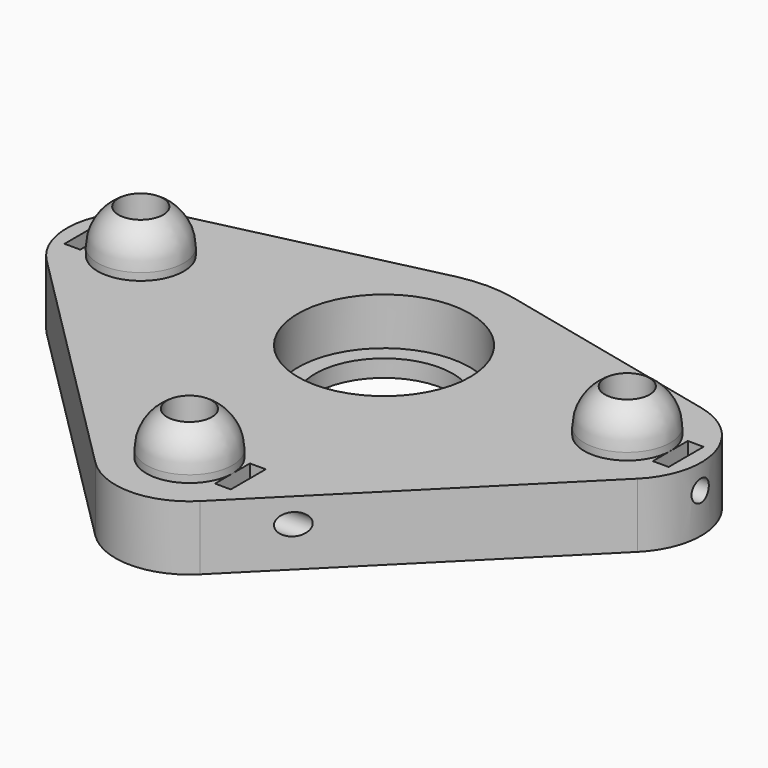
from build123d import *

# Parameters (mm, degrees)
F0_R        = 3.302
F0_R_2      = 12.7
F1_DEPTH    = 9.525
F0_R_3      = 10.16
F2_DEPTH    = 2.54
F5_DEPTH    = 8.636
F6_T1_DEPTH = 2.3368
F6_T3_DEPTH = 2.3368
F6_T5_DEPTH = 2.3368
F3_R        = 6.35
F3_R_2      = 3.302
F7_DEPTH    = 6.35
F11_R       = 1.5875
F12_DEPTH   = 6.35
F9_R        = 1.5875
F13_DEPTH   = 6.35
F10_R       = 1.5875
F14_DEPTH   = 8.382


# Not quite as in the source:
# - a fillet or chamfer that OpenCascade refuses, or shapes differently, is made with other operations: its cross-section is extruded or revolved along the edge and cut away or added
# - a feature names something its author has since deleted; it is built from what else it names


with BuildPart() as f1:
    # F0 (on Top) → F1 (new body)
    with BuildSketch(Plane.XY):
        with BuildLine():
            Line((38.3924752276, 46.5596586637), (4.3105120801, 54.476849111))
            ThreePointArc((4.3105120801, 54.476849111), (0, 54.970934), (-4.3105120801, 54.476849111))
            Line((-4.3105120801, 54.476849111), (-38.3924752276, 46.5596586637))
            ThreePointArc((-38.3924752276, 46.5596586637), (-46.4220600308, 38.9243049052), (-43.6441157783, 28.1978942818))
            Line((-43.6441157783, 28.1978942818), (-7.72300081, -7.7230397182))
            ThreePointArc((-7.72300081, -7.7230397182), (0, -10.922), (7.72300081, -7.7230397182))
            Line((7.72300081, -7.7230397182), (43.6441157783, 28.1978942818))
            ThreePointArc((43.6441157783, 28.1978942818), (46.4220600308, 38.9243049052), (38.3924752276, 46.5596586637))
        make_face()
        Circle(F0_R, mode=Mode.SUBTRACT)
        with Locations((-35.9211149683, 35.920934)):
            Circle(F0_R, mode=Mode.SUBTRACT)
        with Locations((0, 35.920934)):
            Circle(F0_R_2, mode=Mode.SUBTRACT)
        with Locations((35.9211149683, 35.920934)):
            Circle(F0_R, mode=Mode.SUBTRACT)
    extrude(amount=F1_DEPTH)

    # F0 (on Top) → F2 (join)
    with BuildSketch(Plane.XY):
        with Locations((0, 35.920934)):
            Circle(F0_R_2)
        with Locations((0, 35.920934)):
            Circle(F0_R_3, mode=Mode.SUBTRACT)
    extrude(amount=F2_DEPTH)

    # F4 (on face) → F5 (cut)
    with BuildSketch(Plane.XY.offset(9.525)):
        Polygon((-42.2711149683, 32.695134), (-42.2711149683, 35.920934), (-42.2711149683, 39.146734), (-44.6079149683, 39.146734), (-44.6079149683, 32.695134), align=None)
        Polygon((42.2711149683, 39.146734), (42.2711149683, 35.920934), (42.2711149683, 32.695134), (44.6079149683, 32.695134), (44.6079149683, 39.146734), align=None)
        Polygon((6.35, 3.2258), (6.35, 0), (6.35, -3.2258), (8.6868, -3.2258), (8.6868, 3.2258), align=None)
    extrude(amount=-F5_DEPTH, mode=Mode.SUBTRACT)

    # F6: chamfer of 3.175 x 5.499261314 on 6 edges, made by hand

    # F6_s2 → F6_t1 (join)
    with BuildSketch(Plane.YZ.offset(-44.6079149683)):
        Polygon((39.146734, 4.064), (33.647472686, 0.889), (39.146734, 0.889), align=None)
        Polygon((32.695134, 4.064), (38.194395314, 0.889), (32.695134, 0.889), align=None)
    extrude(amount=F6_T1_DEPTH)

    # F6_s4 → F6_t3 (join)
    with BuildSketch(Plane.YZ.offset(6.35)):
        Polygon((3.2258, 4.064), (-2.273461314, 0.889), (3.2258, 0.889), align=None)
        Polygon((-3.2258, 4.064), (2.273461314, 0.889), (-3.2258, 0.889), align=None)
    extrude(amount=F6_T3_DEPTH)

    # F6_s6 → F6_t5 (join)
    with BuildSketch(Plane.YZ.offset(42.2711149683)):
        Polygon((39.146734, 4.064), (33.647472686, 0.889), (39.146734, 0.889), align=None)
        Polygon((32.695134, 4.064), (38.194395314, 0.889), (32.695134, 0.889), align=None)
    extrude(amount=F6_T5_DEPTH)

    # F3 (on face) → F7 (join)
    with BuildSketch(Plane.XY.offset(9.525)):
        with Locations((-35.9211149683, 35.920934)):
            Circle(F3_R)
        with Locations((-35.9211149683, 35.920934)):
            Circle(F3_R_2, mode=Mode.SUBTRACT)
        Circle(F3_R)
        Circle(F3_R_2, mode=Mode.SUBTRACT)
        with Locations((35.9211149683, 35.920934)):
            Circle(F3_R)
        with Locations((35.9211149683, 35.920934)):
            Circle(F3_R_2, mode=Mode.SUBTRACT)
    extrude(amount=F7_DEPTH)

    # F8: fillet of radius 6.096 on 3 edges, made by hand

    # F8_s1 → F8_t2 (revolve, cut)
    with BuildSketch(Plane.XZ.offset(-35.920934)):
        with BuildLine():
            ThreePointArc((-29.5711149683, 10.5957091385), (-30.3878241069, 13.6437091385), (-32.6191149683, 15.875))
            Line((-32.6191149683, 15.875), (-29.5711149683, 15.875))
            Line((-29.5711149683, 15.875), (-29.5711149683, 10.5957091385))
        make_face()
    revolve(axis=Axis((-35.9211149683, 35.920934, 15.875), (0, 0, 1)), mode=Mode.SUBTRACT)

    # F8_s3 → F8_t4 (revolve, cut)
    with BuildSketch(Plane.XZ.offset(-35.920934)):
        with BuildLine():
            ThreePointArc((42.2711149683, 10.5957091385), (41.4544058298, 13.6437091385), (39.2231149683, 15.875))
            Line((39.2231149683, 15.875), (42.2711149683, 15.875))
            Line((42.2711149683, 15.875), (42.2711149683, 10.5957091385))
        make_face()
    revolve(axis=Axis((35.9211149683, 35.920934, 15.875), (0, 0, 1)), mode=Mode.SUBTRACT)

    # F8_s5 → F8_t6 (revolve, cut)
    with BuildSketch(Plane.XZ):
        with BuildLine():
            ThreePointArc((6.35, 10.5957091385), (5.5332908615, 13.6437091385), (3.302, 15.875))
            Line((3.302, 15.875), (6.35, 15.875))
            Line((6.35, 15.875), (6.35, 10.5957091385))
        make_face()
    revolve(axis=Axis((0, 0, 15.875), (0, 0, 1)), mode=Mode.SUBTRACT)

    # F11 (on face) → F12 (cut, symmetric)
    with BuildSketch(Plane(origin=(44.6079149683, 0, 0), x_dir=(0, -1, 0), z_dir=(-1, 0, 0))):
        with Locations((-35.8627085169, 5.8928)):
            Circle(F11_R)
    extrude(amount=F12_DEPTH, both=True, mode=Mode.SUBTRACT)

    # F9 (on face) → F13 (cut, symmetric)
    with BuildSketch(Plane.YZ.offset(-44.6079149683)):
        with Locations((35.8627085169, 5.8928)):
            Circle(F9_R)
    extrude(amount=F13_DEPTH, both=True, mode=Mode.SUBTRACT)

    # F10 (on face) → F14 (cut, symmetric)
    with BuildSketch(Plane(origin=(8.6868, 0, 0), x_dir=(0, -1, 0), z_dir=(-1, 0, 0))):
        with Locations((0.0582254831, 5.8928)):
            Circle(F10_R)
    extrude(amount=F14_DEPTH, both=True, mode=Mode.SUBTRACT)


solid = f1.part
